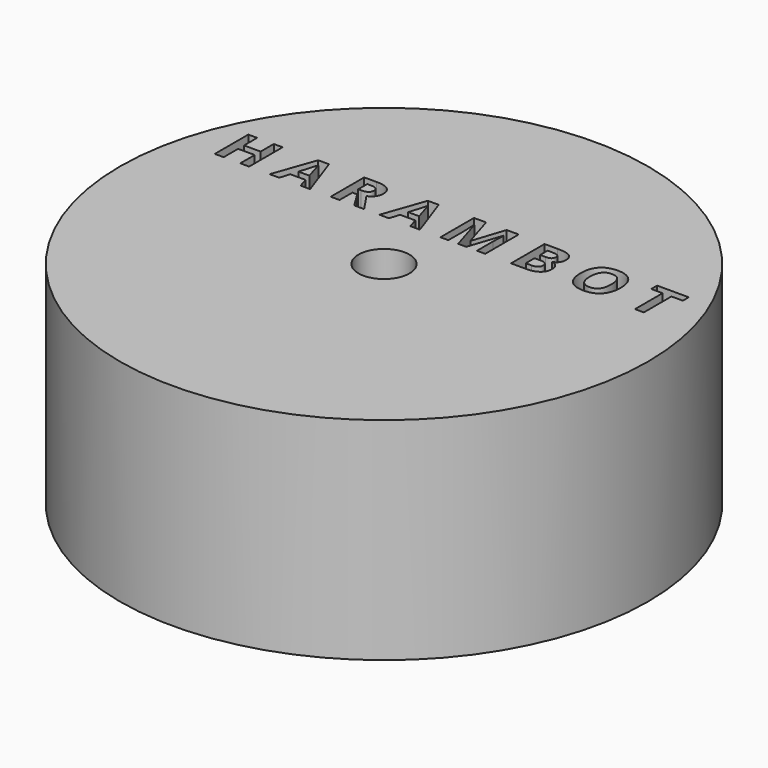
from build123d import *

# Parameters (mm, degrees)
F0_R         = 25
F1_DEPTH     = 20
F3_TEXT_SIZE = 5.5555555556
F4_DEPTH     = 2.5
F2_R         = 2.413
F5_DEPTH     = 20.001


# Not quite as in the source:
# - Text() gives the source's letters only with a copy of the font that has no kerning and outlines rounded to 1/6400 em; it was checked with that copy


with BuildPart() as f1:
    # F0 (on Top) → F1 (new body)
    with BuildSketch(Plane.XY):
        Circle(F0_R)
    extrude(amount=F1_DEPTH)

    # F3 (on face) → F4 (cut)
    with BuildSketch(Plane.XY.offset(20)):
        with Locations((-21.2743055556, 5.9460908819)):
            Text('H A R A M B O T', F3_TEXT_SIZE, font='Open Sans', font_style=FontStyle.BOLD, text_align=(TextAlign.LEFT, TextAlign.BOTTOM))
    extrude(amount=-F4_DEPTH, mode=Mode.SUBTRACT)

    # F2 (on face) → F5 (cut, through all)
    with BuildSketch(Plane.XY.offset(20)):
        Circle(F2_R)
    extrude(amount=-F5_DEPTH, mode=Mode.SUBTRACT)


solid = f1.part
